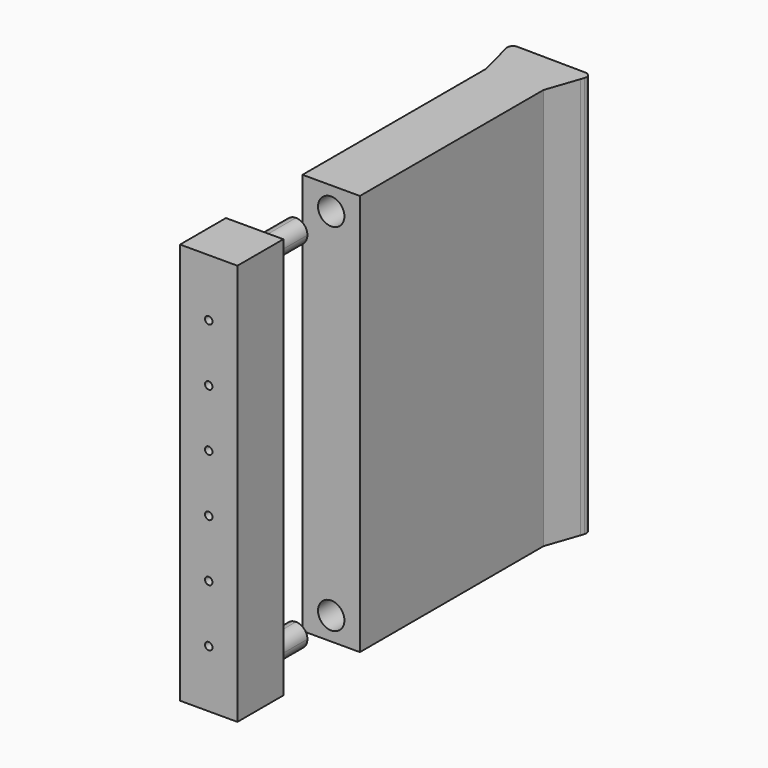
from build123d import *

# Parameters (mm, degrees)
F0_W     = 5
F0_H     = 20
F1_DEPTH = 35
F3_D     = 2.3
F3_DEPTH = 5.3
F3_TIP   = 0.6909897119
F4_W     = 5
F4_H     = 5
F5_DEPTH = 35
F7_DEPTH = 4.5
F8_DEPTH = 4.5
F9_D     = 0.65


with BuildPart() as f1:
    # F0 (on Top) → F1 (new body)
    with BuildSketch(Plane.XY):
        with BuildLine():
            Line((-48.6159127692, 33.1810608496), (-47.8659127692, 30.27632334))
            Line((-47.8659127692, 30.27632334), (-42.8659127692, 30.27632334))
            Line((-42.8659127692, 30.27632334), (-41.8917350471, 33.1137478352))
            Line((-41.8917350471, 33.1137478352), (-41.7914881167, 33.405730591))
            ThreePointArc((-41.7914881167, 33.405730591), (-41.8556853093, 33.8561190265), (-42.2582444333, 34.0680557482))
            Line((-42.2582444333, 34.0680557482), (-42.5669335468, 34.071851532))
            Line((-42.5669335468, 34.071851532), (-47.8659883621, 34.1370111544))
            Line((-47.8659883621, 34.1370111544), (-48.2122020504, 34.1412683576))
            ThreePointArc((-48.2122020504, 34.1412683576), (-48.6117446568, 33.9499167493), (-48.7024727346, 33.5163061541))
            Line((-48.7024727346, 33.5163061541), (-48.6159127692, 33.1810608496))
        make_face()
        with Locations((-45.3659127692, 20.27632334)):
            Rectangle(F0_W, F0_H)
    extrude(amount=F1_DEPTH)

    # F3
    with Locations(Plane.XZ.offset(-10.27632334)):
        with Locations((-45.3659127692, 2), (-45.3659127692, 33)):
            Hole(F3_D / 2, depth=F3_DEPTH)
            with Locations((0, 0, -(F3_DEPTH + F3_TIP / 2))):  # 118° drill point
                Cone(0, F3_D / 2, F3_TIP, mode=Mode.SUBTRACT)


with BuildPart() as f5:
    # F4 (on Top) → F5 (new body)
    with BuildSketch(Plane.XY):
        with Locations((-29.8513197899, 19.5413851738)):
            Rectangle(F4_W, F4_H)
    extrude(amount=F5_DEPTH)

    # F6 (on face) → F7 (join)
    with BuildSketch(Plane(origin=(0, 22.0413851738, 0), x_dir=(-1, 0, 0), z_dir=(0, 1, 0))):
        with BuildLine():
            ThreePointArc((29.8513197899, 3), (29.1448564154, 2.707749603), (28.8513214443, 2.0018190011))
            Line((28.8513214443, 2.0018190011), (29.8513197899, 2))
            Line((29.8513197899, 2), (29.8513197899, 3))
        make_face()
        with BuildLine():
            Line((29.8513197899, 2), (28.8513214443, 2.0018190011))
            ThreePointArc((28.8513214443, 2.0018190011), (29.1435701869, 1.2935366255), (29.8513197899, 1))
            Line((29.8513197899, 1), (29.8513197899, 2))
        make_face()
        with BuildLine():
            ThreePointArc((30.8513197899, 2), (30.5584265711, 2.7071067812), (29.8513197899, 3))
            Line((29.8513197899, 3), (29.8513197899, 2))
            Line((29.8513197899, 2), (29.8513197899, 1))
            ThreePointArc((29.8513197899, 1), (30.5584265711, 1.2928932188), (30.8513197899, 2))
        make_face()
    extrude(amount=F7_DEPTH)

    # F6 (on face) → F8 (join)
    with BuildSketch(Plane(origin=(0, 22.0413851738, 0), x_dir=(-1, 0, 0), z_dir=(0, 1, 0))):
        with BuildLine():
            Line((29.8513197899, 33), (29.8513197899, 34))
            ThreePointArc((29.8513197899, 34), (29.1442130087, 33.7071067812), (28.8513197899, 33))
            Line((28.8513197899, 33), (29.8513197899, 33))
        make_face()
        with BuildLine():
            ThreePointArc((28.8513197899, 33), (29.1442130087, 32.2928932188), (29.8513197899, 32))
            Line((29.8513197899, 32), (29.8513197899, 33))
            Line((29.8513197899, 33), (28.8513197899, 33))
        make_face()
        with BuildLine():
            ThreePointArc((29.8513197899, 32), (30.5584265711, 32.2928932188), (30.8513197899, 33))
            ThreePointArc((30.8513197899, 33), (30.5584265711, 33.7071067812), (29.8513197899, 34))
            Line((29.8513197899, 34), (29.8513197899, 33))
            Line((29.8513197899, 33), (29.8513197899, 32))
        make_face()
    extrude(amount=F8_DEPTH)

    # F9 (through all)
    with Locations(Plane(origin=(0, 22.0413851738, 0), x_dir=(-1, 0, 0), z_dir=(0, 1, 0))):
        with Locations((29.8513197899, 30), (29.8513197899, 25), (29.8513197899, 20), (29.8513197899, 15), (29.8513197899, 10), (29.8513197899, 5)):
            Hole(F9_D / 2)


with BuildPart() as f1_1:
    # F10: moved
    add(f1.part.moved(Location((15.6, 0, 0))))


with BuildPart() as f1_2:
    # F11: moved
    add(f1_1.part.moved(Location((0, 20, 0))))


solid = Compound([f5.part, f1_2.part])
